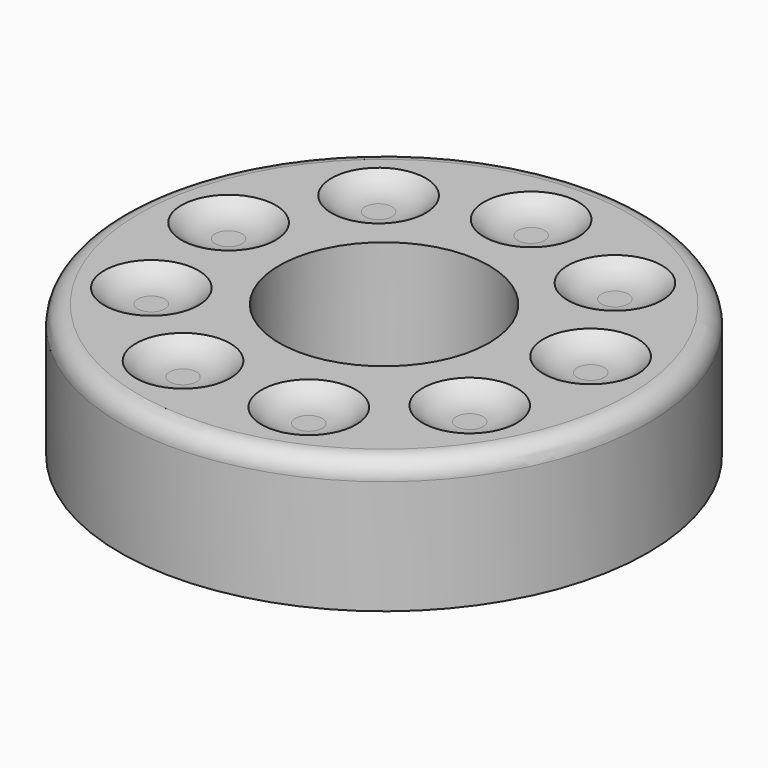
from build123d import *

# Parameters (mm, degrees)
F0_R     = 28
F0_R_2   = 11.125
F1_DEPTH = 14.1
F2_R     = 2
F3_R     = 5
F4_DEPTH = 1.5


# Not quite as in the source:
# - a fillet or chamfer that OpenCascade refuses, or shapes differently, is made with other operations: its cross-section is extruded or revolved along the edge and cut away or added


with BuildPart() as f1:
    # F0 (on Top) → F1 (new body)
    with BuildSketch(Plane.XY):
        Circle(F0_R)
        Circle(F0_R_2, mode=Mode.SUBTRACT)
    extrude(amount=F1_DEPTH)

    # F2
    f2_edges = [f1.edges().sort_by_distance(p)[0] for p in [
        (-28, 0, 14.1),
    ]]
    fillet(f2_edges, radius=F2_R)

    # F3 (on face) → F4 (cut)
    with BuildSketch(Plane.XY.offset(14.1)):
        with Locations((0, 19.5)):
            Circle(F3_R)
        with Locations((-12.5343583889, 14.9378666408)):
            Circle(F3_R)
        with Locations((-19.2037511837, 3.3861394645)):
            Circle(F3_R)
        with Locations((-16.8874953738, -9.75)):
            Circle(F3_R)
        with Locations((-6.6693927949, -18.3240061053)):
            Circle(F3_R)
        with Locations((6.6693927949, -18.3240061053)):
            Circle(F3_R)
        with Locations((16.8874953738, -9.75)):
            Circle(F3_R)
        with Locations((19.2037511837, 3.3861394645)):
            Circle(F3_R)
        with Locations((12.5343583889, 14.9378666408)):
            Circle(F3_R)
    extrude(amount=-F4_DEPTH, mode=Mode.SUBTRACT)

    # F5: fillet of radius 5 on 9 edges, made by hand

    # F5_s1 → F5_t2 (revolve)
    with BuildSketch(Plane.XZ.offset(-19.5)):
        with BuildLine():
            ThreePointArc((5, 14.1), (3.3657774588, 12.9902277714), (1.4292857857, 12.6))
            Line((1.4292857857, 12.6), (5, 12.6))
            Line((5, 12.6), (5, 14.1))
        make_face()
    revolve(axis=Axis((0, 19.5, 12.6), (0, 0, 1)))

    # F5_s3 → F5_t4 (revolve)
    with BuildSketch(Plane.XZ.offset(-14.9378666408)):
        with BuildLine():
            ThreePointArc((-7.5343583889, 14.1), (-9.1685809301, 12.9902277714), (-11.1050726032, 12.6))
            Line((-11.1050726032, 12.6), (-7.5343583889, 12.6))
            Line((-7.5343583889, 12.6), (-7.5343583889, 14.1))
        make_face()
    revolve(axis=Axis((-12.5343583889, 14.9378666408, 12.6), (0, 0, 1)))

    # F5_s5 → F5_t6 (revolve)
    with BuildSketch(Plane.XZ.offset(-3.3861394645)):
        with BuildLine():
            ThreePointArc((-14.2037511837, 14.1), (-15.8379737249, 12.9902277714), (-17.774465398, 12.6))
            Line((-17.774465398, 12.6), (-14.2037511837, 12.6))
            Line((-14.2037511837, 12.6), (-14.2037511837, 14.1))
        make_face()
    revolve(axis=Axis((-19.2037511837, 3.3861394645, 12.6), (0, 0, 1)))

    # F5_s7 → F5_t8 (revolve)
    with BuildSketch(Plane.XZ.offset(9.75)):
        with BuildLine():
            ThreePointArc((-11.8874953738, 14.1), (-13.521717915, 12.9902277714), (-15.4582095881, 12.6))
            Line((-15.4582095881, 12.6), (-11.8874953738, 12.6))
            Line((-11.8874953738, 12.6), (-11.8874953738, 14.1))
        make_face()
    revolve(axis=Axis((-16.8874953738, -9.75, 12.6), (0, 0, 1)))

    # F5_s9 → F5_t10 (revolve)
    with BuildSketch(Plane.XZ.offset(18.3240061053)):
        with BuildLine():
            ThreePointArc((-1.6693927949, 14.1), (-3.303615336, 12.9902277714), (-5.2401070091, 12.6))
            Line((-5.2401070091, 12.6), (-1.6693927949, 12.6))
            Line((-1.6693927949, 12.6), (-1.6693927949, 14.1))
        make_face()
    revolve(axis=Axis((-6.6693927949, -18.3240061053, 12.6), (0, 0, 1)))

    # F5_s11 → F5_t12 (revolve)
    with BuildSketch(Plane.XZ.offset(18.3240061053)):
        with BuildLine():
            ThreePointArc((11.6693927949, 14.1), (10.0351702537, 12.9902277714), (8.0986785806, 12.6))
            Line((8.0986785806, 12.6), (11.6693927949, 12.6))
            Line((11.6693927949, 12.6), (11.6693927949, 14.1))
        make_face()
    revolve(axis=Axis((6.6693927949, -18.3240061053, 12.6), (0, 0, 1)))

    # F5_s13 → F5_t14 (revolve)
    with BuildSketch(Plane.XZ.offset(9.75)):
        with BuildLine():
            ThreePointArc((21.8874953738, 14.1), (20.2532728326, 12.9902277714), (18.3167811595, 12.6))
            Line((18.3167811595, 12.6), (21.8874953738, 12.6))
            Line((21.8874953738, 12.6), (21.8874953738, 14.1))
        make_face()
    revolve(axis=Axis((16.8874953738, -9.75, 12.6), (0, 0, 1)))

    # F5_s15 → F5_t16 (revolve)
    with BuildSketch(Plane.XZ.offset(-3.3861394645)):
        with BuildLine():
            ThreePointArc((24.2037511837, 14.1), (22.5695286426, 12.9902277714), (20.6330369695, 12.6))
            Line((20.6330369695, 12.6), (24.2037511837, 12.6))
            Line((24.2037511837, 12.6), (24.2037511837, 14.1))
        make_face()
    revolve(axis=Axis((19.2037511837, 3.3861394645, 12.6), (0, 0, 1)))

    # F5_s17 → F5_t18 (revolve)
    with BuildSketch(Plane.XZ.offset(-14.9378666408)):
        with BuildLine():
            ThreePointArc((17.5343583889, 14.1), (15.9001358477, 12.9902277714), (13.9636441746, 12.6))
            Line((13.9636441746, 12.6), (17.5343583889, 12.6))
            Line((17.5343583889, 12.6), (17.5343583889, 14.1))
        make_face()
    revolve(axis=Axis((12.5343583889, 14.9378666408, 12.6), (0, 0, 1)))


solid = f1.part
